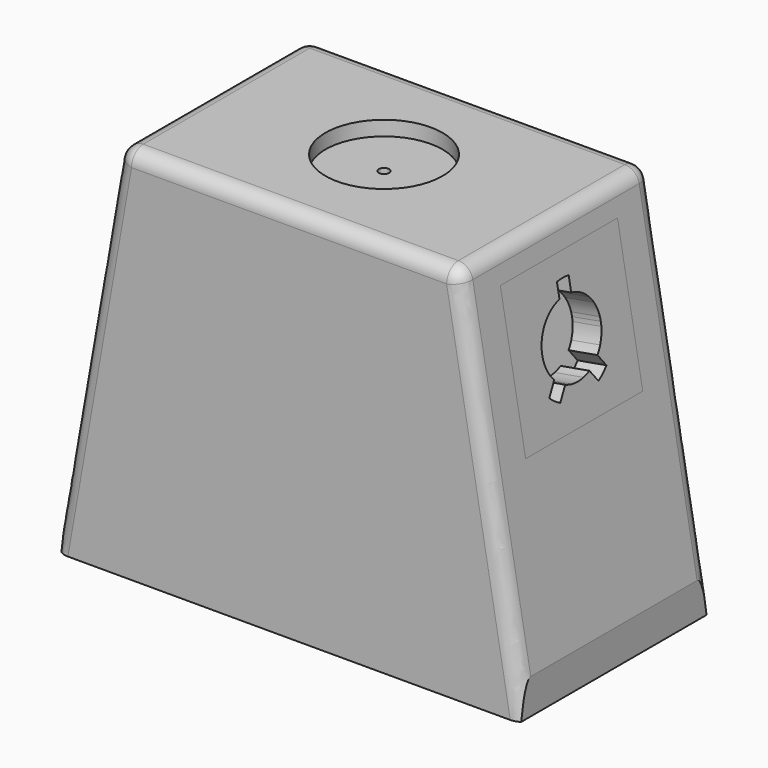
from build123d import *

# Parameters (mm, degrees)
F0_W      = 157
F0_H      = 81
F1_DEPTH  = 12
F1_FACE_W = 157
F1_FACE_H = 81
F3_W      = 116
F3_H      = 81
F5_W      = 49.5
F5_H      = 49.5
F6_DEPTH  = 50
F7_W      = 36
F7_H      = 49.5
F8_DEPTH  = 62.4
F9_W      = 50
F9_H      = 50
F10_DEPTH = 10
F11_W     = 40
F11_H     = 40
F12_DEPTH = 25
F13_W     = 50
F13_H     = 50
F13_W_2   = 40
F13_H_2   = 40
F14_DEPTH = 10
F16_DEPTH = 10
F17_W     = 50
F17_H     = 50
F18_DEPTH = 10
F19_W     = 40
F19_H     = 40
F20_DEPTH = 25
F21_W     = 50
F21_H     = 50
F21_W_2   = 40
F21_H_2   = 40
F22_DEPTH = 10
F24_DEPTH = 25
F25_R     = 20
F26_DEPTH = 5
F27_R     = 5
F28_R     = 1.8
F29_DEPTH = 11
F30_W     = 7.5
F30_H     = 49.5
F31_DEPTH = 23.5
F32_W     = 7.5
F32_H     = 49.5
F33_DEPTH = 23.5


with BuildPart() as f1:
    # F0 (on Top) → F1 (new body)
    with BuildSketch(Plane.XY):
        Rectangle(F0_W, F0_H)
    extrude(amount=F1_DEPTH)

    # F1_face (on face) → F4 section 0
    with BuildSketch(Plane.XY.offset(12)):
        Rectangle(F1_FACE_W, F1_FACE_H)
    # F3 (on offset) → F4 section 1
    with BuildSketch(Plane.XY.offset(129)):
        Rectangle(F3_W, F3_H)
    loft()

    # F5 (on face) → F6 (cut)
    with BuildSketch(Plane(origin=(0, 0, 0), x_dir=(1, 0, 0), z_dir=(0, 0, -1))):
        with Locations((-38.75, 0)):
            Rectangle(F5_W, F5_H)
        with Locations((38.75, 0)):
            Rectangle(F5_W, F5_H)
    extrude(amount=-F6_DEPTH, mode=Mode.SUBTRACT)

    # F7 (on face) → F8 (cut)
    with BuildSketch(Plane(origin=(0, 0, 50), x_dir=(1, 0, 0), z_dir=(0, 0, -1))):
        with Locations((-32, 0)):
            Rectangle(F7_W, F7_H)
        Polygon((-50, -32.5), (50, -32.5), (50, 32.5), (-50, 32.5), (-50, 24.75), (-14, 24.75), (-14, -24.75), (-50, -24.75), align=None)
    extrude(amount=-F8_DEPTH, mode=Mode.SUBTRACT)

    # F9 (on face) → F10 (cut)
    with BuildSketch(Plane(origin=(78.2017825186, 0, 13.7020217233), x_dir=(0, 1, 0), z_dir=(0.9849947084, 0, 0.1725845429))):
        with Locations((0, 82.0544138921)):
            Rectangle(F9_W, F9_H)
    extrude(amount=-F10_DEPTH, mode=Mode.SUBTRACT)

    # F11 (on face) → F12 (cut)
    with BuildSketch(Plane(origin=(68.3518354347, 0, 11.9761762941), x_dir=(0, 1, 0), z_dir=(0.9849947084, 0, 0.1725845429))):
        with Locations((0, 82.0544138921)):
            Rectangle(F11_W, F11_H)
    extrude(amount=-F12_DEPTH, mode=Mode.SUBTRACT)

    # F13 (on face) → F14 (join)
    with BuildSketch(Plane(origin=(68.3518354347, 0, 11.9761762941), x_dir=(0, 1, 0), z_dir=(0.9849947084, 0, 0.1725845429))):
        with Locations((0, 82.0544138921)):
            Rectangle(F13_W, F13_H)
        with Locations((0, 82.0544138921)):
            Rectangle(F13_W_2, F13_H_2, mode=Mode.SUBTRACT)
        with Locations((0, 82.0544138921)):
            Rectangle(F13_W_2, F13_H_2)
    extrude(amount=F14_DEPTH)

    # F15 (on face) → F16 (cut)
    with BuildSketch(Plane(origin=(78.2017825186, 0, 13.7020217233), x_dir=(0, 1, 0), z_dir=(0.9849947084, 0, 0.1725845429))):
        with BuildLine():
            ThreePointArc((-2.5, 94.301862606), (0, 94.5544138921), (2.5, 94.301862606))
            Line((2.5, 94.301862606), (2.5, 99.3749219677))
            ThreePointArc((2.5, 99.3749219677), (0, 99.5544138921), (-2.5, 99.3749219677))
            Line((-2.5, 99.3749219677), (-2.5, 94.301862606))
        make_face()
        with BuildLine():
            Line((2.5, 89.748622735), (2.5, 94.301862606))
            ThreePointArc((2.5, 94.301862606), (0, 94.5544138921), (-2.5, 94.301862606))
            Line((-2.5, 94.301862606), (-2.5, 89.748622735))
            Line((-2.5, 89.748622735), (0, 86.3076679338))
            Line((0, 86.3076679338), (2.5, 89.748622735))
        make_face()
        with BuildLine():
            ThreePointArc((-9.2214122182, 73.6154828755), (-7.3473156537, 71.9417014624), (-5.1763272463, 70.676556614))
            Line((-5.1763272463, 70.676556614), (-2.5, 74.3602050491))
            Line((-2.5, 74.3602050491), (-2.5, 78.6134590909))
            Line((-2.5, 78.6134590909), (-6.5450849719, 77.2991313106))
            Line((-6.5450849719, 77.2991313106), (-9.2214122182, 73.6154828755))
        make_face()
        with BuildLine():
            Line((-8.1581967232, 66.5723653769), (-5.1763272463, 70.676556614))
            ThreePointArc((-5.1763272463, 70.676556614), (-7.3473156537, 71.9417014624), (-9.2214122182, 73.6154828755))
            Line((-9.2214122182, 73.6154828755), (-12.203281695, 69.5112916383))
            ThreePointArc((-12.203281695, 69.5112916383), (-10.2862419151, 67.8966164905), (-8.1581967232, 66.5723653769))
        make_face()
        with BuildLine():
            Line((12.203281695, 69.5112916383), (9.2214122182, 73.6154828755))
            ThreePointArc((9.2214122182, 73.6154828755), (7.3473156537, 71.9417014624), (5.1763272463, 70.676556614))
            Line((5.1763272463, 70.676556614), (8.1581967232, 66.5723653769))
            ThreePointArc((8.1581967232, 66.5723653769), (10.2862419151, 67.8966164905), (12.203281695, 69.5112916383))
        make_face()
        with BuildLine():
            ThreePointArc((5.1763272463, 70.676556614), (7.3473156537, 71.9417014624), (9.2214122182, 73.6154828755))
            Line((9.2214122182, 73.6154828755), (6.5450849719, 77.2991313106))
            Line((6.5450849719, 77.2991313106), (2.5, 78.6134590909))
            Line((2.5, 78.6134590909), (2.5, 74.3602050491))
            Line((2.5, 74.3602050491), (5.1763272463, 70.676556614))
        make_face()
        with BuildLine():
            ThreePointArc((-2.5, 69.8069651781), (0, 69.5544138921), (2.5, 69.8069651781))
            Line((2.5, 69.8069651781), (2.5, 74.3602050491))
            Line((2.5, 74.3602050491), (0, 77.8011598503))
            Line((0, 77.8011598503), (-2.5, 74.3602050491))
            Line((-2.5, 74.3602050491), (-2.5, 69.8069651781))
        make_face()
        with BuildLine():
            ThreePointArc((-5.1763272463, 70.676556614), (-3.8627124297, 70.1662074384), (-2.5, 69.8069651781))
            Line((-2.5, 69.8069651781), (-2.5, 74.3602050491))
            Line((-2.5, 74.3602050491), (-5.1763272463, 70.676556614))
        make_face()
        with BuildLine():
            ThreePointArc((2.5, 69.8069651781), (3.8627124297, 70.1662074384), (5.1763272463, 70.676556614))
            Line((5.1763272463, 70.676556614), (2.5, 74.3602050491))
            Line((2.5, 74.3602050491), (2.5, 69.8069651781))
        make_face()
        with BuildLine():
            ThreePointArc((9.2214122182, 73.6154828755), (10.1127124297, 74.7070982384), (10.8754734214, 75.892102811))
            Line((10.8754734214, 75.892102811), (6.5450849719, 77.2991313106))
            Line((6.5450849719, 77.2991313106), (9.2214122182, 73.6154828755))
        make_face()
        with BuildLine():
            ThreePointArc((10.8754734214, 75.892102811), (11.8882064537, 78.1917014624), (12.4205583933, 80.6473853925))
            Line((12.4205583933, 80.6473853925), (8.0901699437, 82.0544138921))
            Line((8.0901699437, 82.0544138921), (4.0450849719, 80.7400861118))
            Line((4.0450849719, 80.7400861118), (6.5450849719, 77.2991313106))
            Line((6.5450849719, 77.2991313106), (10.8754734214, 75.892102811))
        make_face()
        with BuildLine():
            ThreePointArc((12.4205583933, 80.6473853925), (12.4801237958, 81.3497792052), (12.5, 82.0544138921))
            ThreePointArc((12.5, 82.0544138921), (12.4801237958, 82.7590485789), (12.4205583933, 83.4614423917))
            Line((12.4205583933, 83.4614423917), (8.0901699437, 82.0544138921))
            Line((8.0901699437, 82.0544138921), (12.4205583933, 80.6473853925))
        make_face()
        with BuildLine():
            Line((8.0901699437, 82.0544138921), (12.4205583933, 83.4614423917))
            ThreePointArc((12.4205583933, 83.4614423917), (11.8882064537, 85.9171263217), (10.8754734214, 88.2167249731))
            Line((10.8754734214, 88.2167249731), (6.5450849719, 86.8096964735))
            Line((6.5450849719, 86.8096964735), (4.0450849719, 83.3687416724))
            Line((4.0450849719, 83.3687416724), (8.0901699437, 82.0544138921))
        make_face()
        with BuildLine():
            Line((6.5450849719, 86.8096964735), (9.2214122182, 90.4933449086))
            ThreePointArc((9.2214122182, 90.4933449086), (7.3473156537, 92.1671263217), (5.1763272463, 93.4322711701))
            Line((5.1763272463, 93.4322711701), (2.5, 89.748622735))
            Line((2.5, 89.748622735), (2.5, 85.4953686932))
            Line((2.5, 85.4953686932), (6.5450849719, 86.8096964735))
        make_face()
        with BuildLine():
            Line((6.5450849719, 86.8096964735), (10.8754734214, 88.2167249731))
            ThreePointArc((10.8754734214, 88.2167249731), (10.1127124297, 89.4017295457), (9.2214122182, 90.4933449086))
            Line((9.2214122182, 90.4933449086), (6.5450849719, 86.8096964735))
        make_face()
        with BuildLine():
            Line((2.5, 89.748622735), (5.1763272463, 93.4322711701))
            ThreePointArc((5.1763272463, 93.4322711701), (3.8627124297, 93.9426203457), (2.5, 94.301862606))
            Line((2.5, 94.301862606), (2.5, 89.748622735))
        make_face()
        with BuildLine():
            Line((-2.5, 89.748622735), (-2.5, 94.301862606))
            ThreePointArc((-2.5, 94.301862606), (-3.8627124297, 93.9426203457), (-5.1763272463, 93.4322711701))
            Line((-5.1763272463, 93.4322711701), (-2.5, 89.748622735))
        make_face()
        with BuildLine():
            Line((-2.5, 89.748622735), (-5.1763272463, 93.4322711701))
            ThreePointArc((-5.1763272463, 93.4322711701), (-7.3473156537, 92.1671263217), (-9.2214122182, 90.4933449086))
            Line((-9.2214122182, 90.4933449086), (-6.5450849719, 86.8096964735))
            Line((-6.5450849719, 86.8096964735), (-2.5, 85.4953686932))
            Line((-2.5, 85.4953686932), (-2.5, 89.748622735))
        make_face()
        with BuildLine():
            Line((-6.5450849719, 86.8096964735), (-9.2214122182, 90.4933449086))
            ThreePointArc((-9.2214122182, 90.4933449086), (-10.1127124297, 89.4017295457), (-10.8754734214, 88.2167249731))
            Line((-10.8754734214, 88.2167249731), (-6.5450849719, 86.8096964735))
        make_face()
        with BuildLine():
            Line((-6.5450849719, 86.8096964735), (-10.8754734214, 88.2167249731))
            ThreePointArc((-10.8754734214, 88.2167249731), (-11.8882064537, 85.9171263217), (-12.4205583933, 83.4614423917))
            Line((-12.4205583933, 83.4614423917), (-8.0901699437, 82.0544138921))
            Line((-8.0901699437, 82.0544138921), (-4.0450849719, 83.3687416724))
            Line((-4.0450849719, 83.3687416724), (-6.5450849719, 86.8096964735))
        make_face()
        with BuildLine():
            Line((-8.0901699437, 82.0544138921), (-12.4205583933, 83.4614423917))
            ThreePointArc((-12.4205583933, 83.4614423917), (-12.5, 82.0544138921), (-12.4205583933, 80.6473853925))
            Line((-12.4205583933, 80.6473853925), (-8.0901699437, 82.0544138921))
        make_face()
        with BuildLine():
            ThreePointArc((-10.8754734214, 75.892102811), (-10.1127124297, 74.7070982384), (-9.2214122182, 73.6154828755))
            Line((-9.2214122182, 73.6154828755), (-6.5450849719, 77.2991313106))
            Line((-6.5450849719, 77.2991313106), (-10.8754734214, 75.892102811))
        make_face()
        with BuildLine():
            ThreePointArc((-12.4205583933, 80.6473853925), (-11.8882064537, 78.1917014624), (-10.8754734214, 75.892102811))
            Line((-10.8754734214, 75.892102811), (-6.5450849719, 77.2991313106))
            Line((-6.5450849719, 77.2991313106), (-4.0450849719, 80.7400861118))
            Line((-4.0450849719, 80.7400861118), (-8.0901699437, 82.0544138921))
            Line((-8.0901699437, 82.0544138921), (-12.4205583933, 80.6473853925))
        make_face()
        Polygon((2.5, 78.6134590909), (2.5, 80.238057572), (1.5450849719, 79.9277868712), (0.9549150281, 79.1154876306), align=None)
        Polygon((2.0225424859, 83.5238770228), (1.5450849719, 84.1810409129), (0.7725424859, 84.4320551828), (0, 82.0544138921), align=None)
        Polygon((2.5, 74.3602050491), (2.5, 78.6134590909), (0.9549150281, 79.1154876306), (0, 77.8011598503), align=None)
        Polygon((-2.5, 82.8667131326), (-2.5, 83.8707702121), (-4.0450849719, 83.3687416724), (-3.0901699437, 82.0544138921), align=None)
        Polygon((3.0901699437, 82.0544138921), (4.0450849719, 83.3687416724), (2.5, 83.8707702121), (2.5, 82.8667131326), align=None)
        Polygon((6.5450849719, 77.2991313106), (4.0450849719, 80.7400861118), (2.5, 80.238057572), (2.5, 78.6134590909), align=None)
        Polygon((-0.9549150281, 84.9933401535), (0, 86.3076679338), (-2.5, 89.748622735), (-2.5, 85.4953686932), align=None)
        Polygon((-2.0225424859, 83.5238770228), (-1.5450849719, 84.1810409129), (-2.5, 83.8707702121), (-2.5, 82.8667131326), align=None)
        Polygon((1.5450849719, 84.1810409129), (0.9549150281, 84.9933401535), (0, 84.6830694527), (0.7725424859, 84.4320551828), align=None)
        Polygon((2.0225424859, 80.5849507613), (2.5, 81.2421146515), (2.5, 82.0544138921), (0, 82.0544138921), align=None)
        Polygon((0.9549150281, 84.9933401535), (2.5, 85.4953686932), (2.5, 89.748622735), (0, 86.3076679338), align=None)
        Polygon((-1.5450849719, 79.9277868712), (-2.0225424859, 80.5849507613), (-2.5, 81.2421146515), (-2.5, 80.238057572), align=None)
        Polygon((2.5, 80.238057572), (4.0450849719, 80.7400861118), (3.0901699437, 82.0544138921), (2.5, 81.2421146515), align=None)
        Polygon((0, 79.4257583315), (0.7725424859, 79.6767726013), (0, 82.0544138921), (-0.7725424859, 79.6767726013), align=None)
        Polygon((4.0450849719, 83.3687416724), (6.5450849719, 86.8096964735), (2.5, 85.4953686932), (2.5, 83.8707702121), align=None)
        Polygon((-2.5, 74.3602050491), (0, 77.8011598503), (-0.9549150281, 79.1154876306), (-2.5, 78.6134590909), align=None)
        Polygon((0, 77.8011598503), (0.9549150281, 79.1154876306), (0, 79.4257583315), (-0.9549150281, 79.1154876306), align=None)
        Polygon((0.7725424859, 79.6767726013), (1.5450849719, 79.9277868712), (2.0225424859, 80.5849507613), (0, 82.0544138921), align=None)
        Polygon((2.5, 81.2421146515), (3.0901699437, 82.0544138921), (2.5, 82.8667131326), (2.5, 82.0544138921), align=None)
        Polygon((-2.5, 82.0544138921), (0, 82.0544138921), (-2.0225424859, 83.5238770228), (-2.5, 82.8667131326), align=None)
        Polygon((-2.0225424859, 80.5849507613), (0, 82.0544138921), (-2.5, 82.0544138921), (-2.5, 81.2421146515), align=None)
        Polygon((-2.5, 81.2421146515), (-2.5, 82.0544138921), (-2.5, 82.8667131326), (-3.0901699437, 82.0544138921), align=None)
        Polygon((-6.5450849719, 77.2991313106), (-2.5, 78.6134590909), (-2.5, 80.238057572), (-4.0450849719, 80.7400861118), align=None)
        Polygon((-2.5, 78.6134590909), (-0.9549150281, 79.1154876306), (-1.5450849719, 79.9277868712), (-2.5, 80.238057572), align=None)
        Polygon((4.0450849719, 80.7400861118), (8.0901699437, 82.0544138921), (4.0450849719, 83.3687416724), (3.0901699437, 82.0544138921), align=None)
        Polygon((-0.9549150281, 79.1154876306), (0, 79.4257583315), (-0.7725424859, 79.6767726013), (-1.5450849719, 79.9277868712), align=None)
        Polygon((0, 84.6830694527), (0.9549150281, 84.9933401535), (0, 86.3076679338), (-0.9549150281, 84.9933401535), align=None)
        Polygon((-0.7725424859, 79.6767726013), (0, 82.0544138921), (-2.0225424859, 80.5849507613), (-1.5450849719, 79.9277868712), align=None)
        Polygon((0.7725424859, 84.4320551828), (0, 84.6830694527), (-0.7725424859, 84.4320551828), (0, 82.0544138921), align=None)
        Polygon((2.5, 82.0544138921), (2.5, 82.8667131326), (2.0225424859, 83.5238770228), (0, 82.0544138921), align=None)
        Polygon((-2.5, 80.238057572), (-2.5, 81.2421146515), (-3.0901699437, 82.0544138921), (-4.0450849719, 80.7400861118), align=None)
        Polygon((-2.5, 83.8707702121), (-2.5, 85.4953686932), (-6.5450849719, 86.8096964735), (-4.0450849719, 83.3687416724), align=None)
        Polygon((-1.5450849719, 84.1810409129), (-0.9549150281, 84.9933401535), (-2.5, 85.4953686932), (-2.5, 83.8707702121), align=None)
        Polygon((1.5450849719, 79.9277868712), (2.5, 80.238057572), (2.5, 81.2421146515), (2.0225424859, 80.5849507613), align=None)
        Polygon((0, 82.0544138921), (-0.7725424859, 84.4320551828), (-1.5450849719, 84.1810409129), (-2.0225424859, 83.5238770228), align=None)
        Polygon((2.5, 83.8707702121), (2.5, 85.4953686932), (0.9549150281, 84.9933401535), (1.5450849719, 84.1810409129), align=None)
        Polygon((2.5, 82.8667131326), (2.5, 83.8707702121), (1.5450849719, 84.1810409129), (2.0225424859, 83.5238770228), align=None)
        Polygon((-0.7725424859, 84.4320551828), (0, 84.6830694527), (-0.9549150281, 84.9933401535), (-1.5450849719, 84.1810409129), align=None)
        Polygon((0.9549150281, 79.1154876306), (1.5450849719, 79.9277868712), (0.7725424859, 79.6767726013), (0, 79.4257583315), align=None)
        Polygon((-3.0901699437, 82.0544138921), (-4.0450849719, 83.3687416724), (-8.0901699437, 82.0544138921), (-4.0450849719, 80.7400861118), align=None)
    extrude(amount=-F16_DEPTH, mode=Mode.SUBTRACT)

    # F17 (on face) → F18 (cut)
    with BuildSketch(Plane(origin=(-78.2017825186, 0, 13.7020217233), x_dir=(0, -1, 0), z_dir=(-0.9849947084, 0, 0.1725845429))):
        with Locations((0, 82.0544138921)):
            Rectangle(F17_W, F17_H)
    extrude(amount=-F18_DEPTH, mode=Mode.SUBTRACT)

    # F19 (on face) → F20 (cut)
    with BuildSketch(Plane(origin=(-68.3518354347, 0, 11.9761762941), x_dir=(0, -1, 0), z_dir=(-0.9849947084, 0, 0.1725845429))):
        with Locations((0, 82.0544138921)):
            Rectangle(F19_W, F19_H)
    extrude(amount=-F20_DEPTH, mode=Mode.SUBTRACT)

    # F21 (on face) → F22 (join)
    with BuildSketch(Plane(origin=(-68.3518354347, 0, 11.9761762941), x_dir=(0, -1, 0), z_dir=(-0.9849947084, 0, 0.1725845429))):
        with Locations((0, 82.0544138921)):
            Rectangle(F21_W, F21_H)
        with Locations((0, 82.0544138921)):
            Rectangle(F21_W_2, F21_H_2, mode=Mode.SUBTRACT)
        with Locations((0, 82.0544138921)):
            Rectangle(F21_W_2, F21_H_2)
    extrude(amount=F22_DEPTH)

    # F23 (on face) → F24 (cut)
    with BuildSketch(Plane(origin=(-78.2017825186, 0, 13.7020217233), x_dir=(0, -1, 0), z_dir=(-0.9849947084, 0, 0.1725845429))):
        with BuildLine():
            Line((2.5, 94.301862606), (2.5, 99.3749219677))
            ThreePointArc((2.5, 99.3749219677), (0, 99.5544138921), (-2.5, 99.3749219677))
            Line((-2.5, 99.3749219677), (-2.5, 94.301862606))
            ThreePointArc((-2.5, 94.301862606), (0, 94.5544138921), (2.5, 94.301862606))
        make_face()
        with BuildLine():
            Line((2.5, 89.748622735), (2.5, 94.301862606))
            ThreePointArc((2.5, 94.301862606), (0, 94.5544138921), (-2.5, 94.301862606))
            Line((-2.5, 94.301862606), (-2.5, 89.748622735))
            Line((-2.5, 89.748622735), (0, 86.3076679338))
            Line((0, 86.3076679338), (2.5, 89.748622735))
        make_face()
        with BuildLine():
            ThreePointArc((-12.203281695, 69.5112916383), (-10.2862419151, 67.8966164905), (-8.1581967232, 66.5723653769))
            Line((-8.1581967232, 66.5723653769), (-5.1763272463, 70.676556614))
            ThreePointArc((-5.1763272463, 70.676556614), (-7.3473156537, 71.9417014624), (-9.2214122182, 73.6154828755))
            Line((-9.2214122182, 73.6154828755), (-12.203281695, 69.5112916383))
        make_face()
        with BuildLine():
            ThreePointArc((8.1581967232, 66.5723653769), (10.2862419151, 67.8966164905), (12.203281695, 69.5112916383))
            Line((12.203281695, 69.5112916383), (9.2214122182, 73.6154828755))
            ThreePointArc((9.2214122182, 73.6154828755), (7.3473156537, 71.9417014624), (5.1763272463, 70.676556614))
            Line((5.1763272463, 70.676556614), (8.1581967232, 66.5723653769))
        make_face()
        with BuildLine():
            ThreePointArc((-9.2214122182, 73.6154828755), (-7.3473156537, 71.9417014624), (-5.1763272463, 70.676556614))
            Line((-5.1763272463, 70.676556614), (-2.5, 74.3602050491))
            Line((-2.5, 74.3602050491), (-2.5, 78.6134590909))
            Line((-2.5, 78.6134590909), (-6.5450849719, 77.2991313106))
            Line((-6.5450849719, 77.2991313106), (-9.2214122182, 73.6154828755))
        make_face()
        with BuildLine():
            ThreePointArc((5.1763272463, 70.676556614), (7.3473156537, 71.9417014624), (9.2214122182, 73.6154828755))
            Line((9.2214122182, 73.6154828755), (6.5450849719, 77.2991313106))
            Line((6.5450849719, 77.2991313106), (2.5, 78.6134590909))
            Line((2.5, 78.6134590909), (2.5, 74.3602050491))
            Line((2.5, 74.3602050491), (5.1763272463, 70.676556614))
        make_face()
        with BuildLine():
            ThreePointArc((2.5, 69.8069651781), (3.8627124297, 70.1662074384), (5.1763272463, 70.676556614))
            Line((5.1763272463, 70.676556614), (2.5, 74.3602050491))
            Line((2.5, 74.3602050491), (2.5, 69.8069651781))
        make_face()
        with BuildLine():
            ThreePointArc((-5.1763272463, 70.676556614), (-3.8627124297, 70.1662074384), (-2.5, 69.8069651781))
            Line((-2.5, 69.8069651781), (-2.5, 74.3602050491))
            Line((-2.5, 74.3602050491), (-5.1763272463, 70.676556614))
        make_face()
        with BuildLine():
            ThreePointArc((-2.5, 69.8069651781), (0, 69.5544138921), (2.5, 69.8069651781))
            Line((2.5, 69.8069651781), (2.5, 74.3602050491))
            Line((2.5, 74.3602050491), (0, 77.8011598503))
            Line((0, 77.8011598503), (-2.5, 74.3602050491))
            Line((-2.5, 74.3602050491), (-2.5, 69.8069651781))
        make_face()
        with BuildLine():
            ThreePointArc((-10.8754734214, 75.892102811), (-10.1127124297, 74.7070982384), (-9.2214122182, 73.6154828755))
            Line((-9.2214122182, 73.6154828755), (-6.5450849719, 77.2991313106))
            Line((-6.5450849719, 77.2991313106), (-10.8754734214, 75.892102811))
        make_face()
        with BuildLine():
            Line((-8.0901699437, 82.0544138921), (-12.4205583933, 83.4614423917))
            ThreePointArc((-12.4205583933, 83.4614423917), (-12.5, 82.0544138921), (-12.4205583933, 80.6473853925))
            Line((-12.4205583933, 80.6473853925), (-8.0901699437, 82.0544138921))
        make_face()
        with BuildLine():
            ThreePointArc((-12.4205583933, 80.6473853925), (-11.8882064537, 78.1917014624), (-10.8754734214, 75.892102811))
            Line((-10.8754734214, 75.892102811), (-6.5450849719, 77.2991313106))
            Line((-6.5450849719, 77.2991313106), (-4.0450849719, 80.7400861118))
            Line((-4.0450849719, 80.7400861118), (-8.0901699437, 82.0544138921))
            Line((-8.0901699437, 82.0544138921), (-12.4205583933, 80.6473853925))
        make_face()
        with BuildLine():
            Line((-6.5450849719, 86.8096964735), (-9.2214122182, 90.4933449086))
            ThreePointArc((-9.2214122182, 90.4933449086), (-10.1127124297, 89.4017295457), (-10.8754734214, 88.2167249731))
            Line((-10.8754734214, 88.2167249731), (-6.5450849719, 86.8096964735))
        make_face()
        with BuildLine():
            Line((-6.5450849719, 86.8096964735), (-10.8754734214, 88.2167249731))
            ThreePointArc((-10.8754734214, 88.2167249731), (-11.8882064537, 85.9171263217), (-12.4205583933, 83.4614423917))
            Line((-12.4205583933, 83.4614423917), (-8.0901699437, 82.0544138921))
            Line((-8.0901699437, 82.0544138921), (-4.0450849719, 83.3687416724))
            Line((-4.0450849719, 83.3687416724), (-6.5450849719, 86.8096964735))
        make_face()
        with BuildLine():
            Line((-2.5, 89.748622735), (-5.1763272463, 93.4322711701))
            ThreePointArc((-5.1763272463, 93.4322711701), (-7.3473156537, 92.1671263217), (-9.2214122182, 90.4933449086))
            Line((-9.2214122182, 90.4933449086), (-6.5450849719, 86.8096964735))
            Line((-6.5450849719, 86.8096964735), (-2.5, 85.4953686932))
            Line((-2.5, 85.4953686932), (-2.5, 89.748622735))
        make_face()
        with BuildLine():
            Line((-2.5, 89.748622735), (-2.5, 94.301862606))
            ThreePointArc((-2.5, 94.301862606), (-3.8627124297, 93.9426203457), (-5.1763272463, 93.4322711701))
            Line((-5.1763272463, 93.4322711701), (-2.5, 89.748622735))
        make_face()
        with BuildLine():
            Line((6.5450849719, 86.8096964735), (9.2214122182, 90.4933449086))
            ThreePointArc((9.2214122182, 90.4933449086), (7.3473156537, 92.1671263217), (5.1763272463, 93.4322711701))
            Line((5.1763272463, 93.4322711701), (2.5, 89.748622735))
            Line((2.5, 89.748622735), (2.5, 85.4953686932))
            Line((2.5, 85.4953686932), (6.5450849719, 86.8096964735))
        make_face()
        with BuildLine():
            Line((2.5, 89.748622735), (5.1763272463, 93.4322711701))
            ThreePointArc((5.1763272463, 93.4322711701), (3.8627124297, 93.9426203457), (2.5, 94.301862606))
            Line((2.5, 94.301862606), (2.5, 89.748622735))
        make_face()
        with BuildLine():
            Line((8.0901699437, 82.0544138921), (12.4205583933, 83.4614423917))
            ThreePointArc((12.4205583933, 83.4614423917), (11.8882064537, 85.9171263217), (10.8754734214, 88.2167249731))
            Line((10.8754734214, 88.2167249731), (6.5450849719, 86.8096964735))
            Line((6.5450849719, 86.8096964735), (4.0450849719, 83.3687416724))
            Line((4.0450849719, 83.3687416724), (8.0901699437, 82.0544138921))
        make_face()
        with BuildLine():
            Line((6.5450849719, 86.8096964735), (10.8754734214, 88.2167249731))
            ThreePointArc((10.8754734214, 88.2167249731), (10.1127124297, 89.4017295457), (9.2214122182, 90.4933449086))
            Line((9.2214122182, 90.4933449086), (6.5450849719, 86.8096964735))
        make_face()
        with BuildLine():
            ThreePointArc((10.8754734214, 75.892102811), (11.8882064537, 78.1917014624), (12.4205583933, 80.6473853925))
            Line((12.4205583933, 80.6473853925), (8.0901699437, 82.0544138921))
            Line((8.0901699437, 82.0544138921), (4.0450849719, 80.7400861118))
            Line((4.0450849719, 80.7400861118), (6.5450849719, 77.2991313106))
            Line((6.5450849719, 77.2991313106), (10.8754734214, 75.892102811))
        make_face()
        with BuildLine():
            ThreePointArc((12.5, 82.0544138921), (12.4801237958, 82.7590485789), (12.4205583933, 83.4614423917))
            Line((12.4205583933, 83.4614423917), (8.0901699437, 82.0544138921))
            Line((8.0901699437, 82.0544138921), (12.4205583933, 80.6473853925))
            ThreePointArc((12.4205583933, 80.6473853925), (12.4801237958, 81.3497792052), (12.5, 82.0544138921))
        make_face()
        with BuildLine():
            ThreePointArc((9.2214122182, 73.6154828755), (10.1127124297, 74.7070982384), (10.8754734214, 75.892102811))
            Line((10.8754734214, 75.892102811), (6.5450849719, 77.2991313106))
            Line((6.5450849719, 77.2991313106), (9.2214122182, 73.6154828755))
        make_face()
        Polygon((0.7725424859, 84.4320551828), (0, 84.6830694527), (-0.7725424859, 84.4320551828), (0, 82.0544138921), align=None)
        Polygon((0, 77.8011598503), (0.9549150281, 79.1154876306), (0, 79.4257583315), (-0.9549150281, 79.1154876306), align=None)
        Polygon((2.0225424859, 83.5238770228), (1.5450849719, 84.1810409129), (0.7725424859, 84.4320551828), (0, 82.0544138921), align=None)
        Polygon((-0.7725424859, 79.6767726013), (0, 82.0544138921), (-2.0225424859, 80.5849507613), (-1.5450849719, 79.9277868712), align=None)
        Polygon((-2.5, 81.2421146515), (-2.5, 82.0544138921), (-2.5, 82.8667131326), (-3.0901699437, 82.0544138921), align=None)
        Polygon((2.5, 78.6134590909), (2.5, 80.238057572), (1.5450849719, 79.9277868712), (0.9549150281, 79.1154876306), align=None)
        Polygon((-0.9549150281, 84.9933401535), (0, 86.3076679338), (-2.5, 89.748622735), (-2.5, 85.4953686932), align=None)
        Polygon((-2.0225424859, 80.5849507613), (0, 82.0544138921), (-2.5, 82.0544138921), (-2.5, 81.2421146515), align=None)
        Polygon((-2.5, 78.6134590909), (-0.9549150281, 79.1154876306), (-1.5450849719, 79.9277868712), (-2.5, 80.238057572), align=None)
        Polygon((4.0450849719, 80.7400861118), (8.0901699437, 82.0544138921), (4.0450849719, 83.3687416724), (3.0901699437, 82.0544138921), align=None)
        Polygon((0, 84.6830694527), (0.9549150281, 84.9933401535), (0, 86.3076679338), (-0.9549150281, 84.9933401535), align=None)
        Polygon((-1.5450849719, 79.9277868712), (-2.0225424859, 80.5849507613), (-2.5, 81.2421146515), (-2.5, 80.238057572), align=None)
        Polygon((-2.5, 83.8707702121), (-2.5, 85.4953686932), (-6.5450849719, 86.8096964735), (-4.0450849719, 83.3687416724), align=None)
        Polygon((-6.5450849719, 77.2991313106), (-2.5, 78.6134590909), (-2.5, 80.238057572), (-4.0450849719, 80.7400861118), align=None)
        Polygon((2.5, 83.8707702121), (2.5, 85.4953686932), (0.9549150281, 84.9933401535), (1.5450849719, 84.1810409129), align=None)
        Polygon((2.5, 82.0544138921), (2.5, 82.8667131326), (2.0225424859, 83.5238770228), (0, 82.0544138921), align=None)
        Polygon((-2.5, 74.3602050491), (0, 77.8011598503), (-0.9549150281, 79.1154876306), (-2.5, 78.6134590909), align=None)
        Polygon((3.0901699437, 82.0544138921), (4.0450849719, 83.3687416724), (2.5, 83.8707702121), (2.5, 82.8667131326), align=None)
        Polygon((6.5450849719, 77.2991313106), (4.0450849719, 80.7400861118), (2.5, 80.238057572), (2.5, 78.6134590909), align=None)
        Polygon((2.5, 81.2421146515), (3.0901699437, 82.0544138921), (2.5, 82.8667131326), (2.5, 82.0544138921), align=None)
        Polygon((0, 82.0544138921), (-0.7725424859, 84.4320551828), (-1.5450849719, 84.1810409129), (-2.0225424859, 83.5238770228), align=None)
        Polygon((-2.5, 82.0544138921), (0, 82.0544138921), (-2.0225424859, 83.5238770228), (-2.5, 82.8667131326), align=None)
        Polygon((-2.5, 80.238057572), (-2.5, 81.2421146515), (-3.0901699437, 82.0544138921), (-4.0450849719, 80.7400861118), align=None)
        Polygon((1.5450849719, 79.9277868712), (2.5, 80.238057572), (2.5, 81.2421146515), (2.0225424859, 80.5849507613), align=None)
        Polygon((0.7725424859, 79.6767726013), (1.5450849719, 79.9277868712), (2.0225424859, 80.5849507613), (0, 82.0544138921), align=None)
        Polygon((0.9549150281, 84.9933401535), (2.5, 85.4953686932), (2.5, 89.748622735), (0, 86.3076679338), align=None)
        Polygon((2.0225424859, 80.5849507613), (2.5, 81.2421146515), (2.5, 82.0544138921), (0, 82.0544138921), align=None)
        Polygon((2.5, 74.3602050491), (2.5, 78.6134590909), (0.9549150281, 79.1154876306), (0, 77.8011598503), align=None)
        Polygon((4.0450849719, 83.3687416724), (6.5450849719, 86.8096964735), (2.5, 85.4953686932), (2.5, 83.8707702121), align=None)
        Polygon((0, 79.4257583315), (0.7725424859, 79.6767726013), (0, 82.0544138921), (-0.7725424859, 79.6767726013), align=None)
        Polygon((2.5, 80.238057572), (4.0450849719, 80.7400861118), (3.0901699437, 82.0544138921), (2.5, 81.2421146515), align=None)
        Polygon((-2.0225424859, 83.5238770228), (-1.5450849719, 84.1810409129), (-2.5, 83.8707702121), (-2.5, 82.8667131326), align=None)
        Polygon((1.5450849719, 84.1810409129), (0.9549150281, 84.9933401535), (0, 84.6830694527), (0.7725424859, 84.4320551828), align=None)
        Polygon((-1.5450849719, 84.1810409129), (-0.9549150281, 84.9933401535), (-2.5, 85.4953686932), (-2.5, 83.8707702121), align=None)
        Polygon((-0.9549150281, 79.1154876306), (0, 79.4257583315), (-0.7725424859, 79.6767726013), (-1.5450849719, 79.9277868712), align=None)
        Polygon((-2.5, 82.8667131326), (-2.5, 83.8707702121), (-4.0450849719, 83.3687416724), (-3.0901699437, 82.0544138921), align=None)
        Polygon((2.5, 82.8667131326), (2.5, 83.8707702121), (1.5450849719, 84.1810409129), (2.0225424859, 83.5238770228), align=None)
        Polygon((0.9549150281, 79.1154876306), (1.5450849719, 79.9277868712), (0.7725424859, 79.6767726013), (0, 79.4257583315), align=None)
        Polygon((-0.7725424859, 84.4320551828), (0, 84.6830694527), (-0.9549150281, 84.9933401535), (-1.5450849719, 84.1810409129), align=None)
        Polygon((-3.0901699437, 82.0544138921), (-4.0450849719, 83.3687416724), (-8.0901699437, 82.0544138921), (-4.0450849719, 80.7400861118), align=None)
    extrude(amount=-F24_DEPTH, mode=Mode.SUBTRACT)

    # F25 (on face) → F26 (cut)
    with BuildSketch(Plane.XY.offset(129)):
        Circle(F25_R)
    extrude(amount=-F26_DEPTH, mode=Mode.SUBTRACT)

    # F27
    f27_edges = [f1.edges().sort_by_distance(p)[0] for p in [
        (0, 40.5, 129),
        (-58, 0, 129),
        (0, -40.5, 129),
        (58, 0, 129),
        (-68.25, -40.5, 70.5),
        (68.25, -40.5, 70.5),
        (-68.25, 40.5, 70.5),
        (68.25, 40.5, 70.5),
    ]]
    fillet(f27_edges, radius=F27_R)

    # F28 (on face) → F29 (cut)
    with BuildSketch(Plane.XY.offset(124)):
        Circle(F28_R)
    extrude(amount=-F29_DEPTH, mode=Mode.SUBTRACT)

    # F30 (on face) → F31 (cut)
    with BuildSketch(Plane(origin=(0, 0, 50), x_dir=(1, 0, 0), z_dir=(0, 0, -1))):
        with Locations((-53.75, 0)):
            Rectangle(F30_W, F30_H)
    extrude(amount=-F31_DEPTH, mode=Mode.SUBTRACT)

    # F32 (on face) → F33 (cut)
    with BuildSketch(Plane(origin=(0, 0, 50), x_dir=(1, 0, 0), z_dir=(0, 0, -1))):
        with Locations((53.75, 0)):
            Rectangle(F32_W, F32_H)
    extrude(amount=-F33_DEPTH, mode=Mode.SUBTRACT)


solid = f1.part
